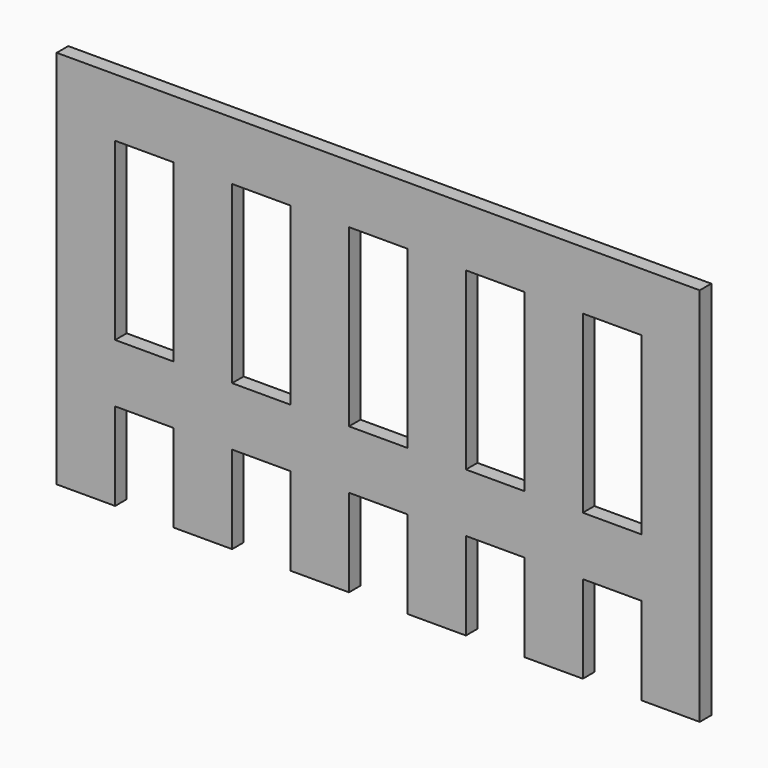
from build123d import *

# Parameters (mm, degrees)
F0_W     = 102.730258709
F0_H     = 102.730258709
F0_H_2   = 308.1907761271
F0_H_3   = 154.0953880636
F1_DEPTH = 25.4


# Not quite as in the source:
# - a feature names something its author has since deleted; it is built from what else it names


with BuildPart() as f1:
    # F0 (on Front) → F1 (new body)
    with BuildSketch(Plane.XZ):
        with Locations((-770.1755237305, 217.3844415066)):
            Rectangle(F0_W, F0_H)
        with Locations((-770.1755237305, 11.9239240885)):
            Rectangle(F0_W, F0_H_2)
        with Locations((-770.1755237305, -193.5365933296)):
            Rectangle(F0_W, F0_H)
        with Locations((-770.1755237305, -321.9494167159)):
            Rectangle(F0_W, F0_H_3)
        with Locations((-564.7150063124, -193.5365933296)):
            Rectangle(F0_W, F0_H)
        with Locations((-564.7150063124, 11.9239240885)):
            Rectangle(F0_W, F0_H_2)
        with Locations((-564.7150063124, 217.3844415066)):
            Rectangle(F0_W, F0_H)
        with Locations((-359.2544888943, 217.3844415066)):
            Rectangle(F0_W, F0_H)
        with Locations((-359.2544888943, 11.9239240885)):
            Rectangle(F0_W, F0_H_2)
        with Locations((-359.2544888943, -321.9494167159)):
            Rectangle(F0_W, F0_H_3)
        with Locations((-564.7150063124, -321.9494167159)):
            Rectangle(F0_W, F0_H_3)
        with Locations((-359.2544888943, -193.5365933296)):
            Rectangle(F0_W, F0_H)
        with Locations((-153.7939714763, -193.5365933296)):
            Rectangle(F0_W, F0_H)
        with Locations((-153.7939714763, 217.3844415066)):
            Rectangle(F0_W, F0_H)
        with Locations((-153.7939714763, -321.9494167159)):
            Rectangle(F0_W, F0_H_3)
        with Locations((51.6665459418, -321.9494167159)):
            Rectangle(F0_W, F0_H_3)
        with Locations((51.6665459418, -193.5365933296)):
            Rectangle(F0_W, F0_H)
        with Locations((51.6665459418, 11.9239240885)):
            Rectangle(F0_W, F0_H_2)
        with Locations((-153.7939714763, 11.9239240885)):
            Rectangle(F0_W, F0_H_2)
        with Locations((51.6665459418, 217.3844415066)):
            Rectangle(F0_W, F0_H)
        with Locations((257.1270633599, 217.3844415066)):
            Rectangle(F0_W, F0_H)
        with Locations((257.1270633599, 11.9239240885)):
            Rectangle(F0_W, F0_H_2)
        with Locations((257.1270633599, -193.5365933296)):
            Rectangle(F0_W, F0_H)
        with Locations((257.1270633599, -321.9494167159)):
            Rectangle(F0_W, F0_H_3)
        with Locations((-667.4452650214, 217.3844415066)):
            Rectangle(F0_W, F0_H)
        with Locations((-667.4452650214, -193.5365933296)):
            Rectangle(F0_W, F0_H)
        with Locations((-461.9847476034, -193.5365933296)):
            Rectangle(F0_W, F0_H)
        with Locations((-461.9847476034, 217.3844415066)):
            Rectangle(F0_W, F0_H)
        with Locations((-256.5242301853, 217.3844415066)):
            Rectangle(F0_W, F0_H)
        with Locations((-256.5242301853, -193.5365933296)):
            Rectangle(F0_W, F0_H)
        with Locations((-51.0637127672, -193.5365933296)):
            Rectangle(F0_W, F0_H)
        with Locations((-51.0637127672, 217.3844415066)):
            Rectangle(F0_W, F0_H)
        with Locations((154.3968046508, 217.3844415066)):
            Rectangle(F0_W, F0_H)
        with Locations((154.3968046508, -193.5365933296)):
            Rectangle(F0_W, F0_H)
    extrude(amount=F1_DEPTH)


solid = f1.part
